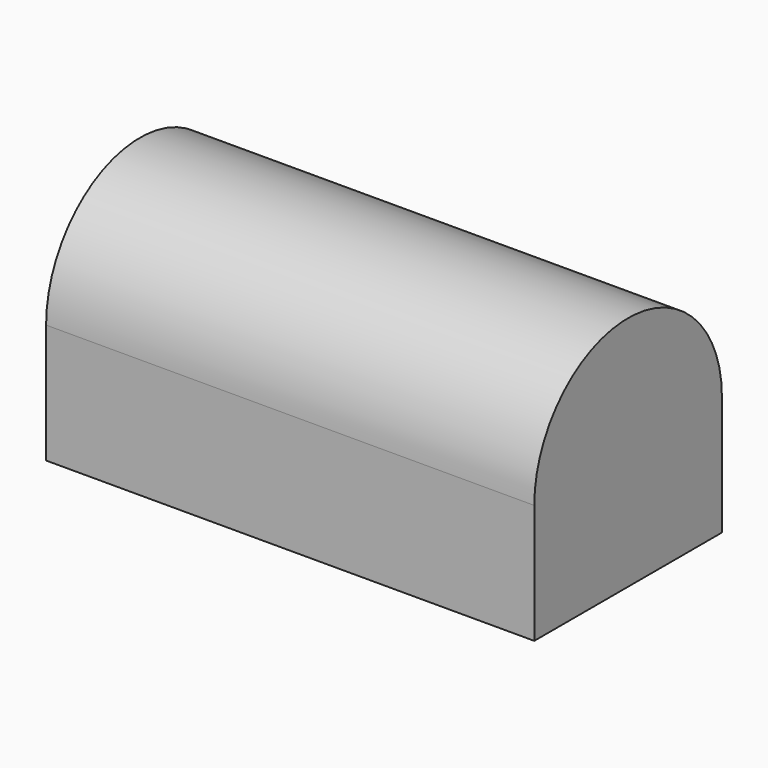
from build123d import *

# Parameters (mm, degrees)
F0_W     = 61.4
F0_H     = 29.5
F1_DEPTH = 30
F3_DEPTH = 61.4


# Not quite as in the source:
# - a feature names something its author has since deleted; it is built from what else it names


with BuildPart() as f1:
    # F0 (on Top) → F1 (new body)
    with BuildSketch(Plane.XY):
        with Locations((1.9898619503, 2.1330590255)):
            Rectangle(F0_W, F0_H)
    extrude(amount=F1_DEPTH)

    # F2 (on face) → F3 (cut, through all)
    with BuildSketch(Plane.YZ.offset(32.6898619503)):
        with BuildLine():
            Line((9.1330590255, 30), (-4.8669409745, 30))
            Line((-4.8669409745, 30), (-12.6169409745, 30))
            Line((-12.6169409745, 30), (-12.6169409745, 15))
            ThreePointArc((-12.6169409745, 15), (2.1330590255, 29.75), (16.8830590255, 15))
            Line((16.8830590255, 15), (16.8830590255, 30))
            Line((16.8830590255, 30), (9.1330590255, 30))
        make_face()
    extrude(amount=-F3_DEPTH, mode=Mode.SUBTRACT)


solid = f1.part
